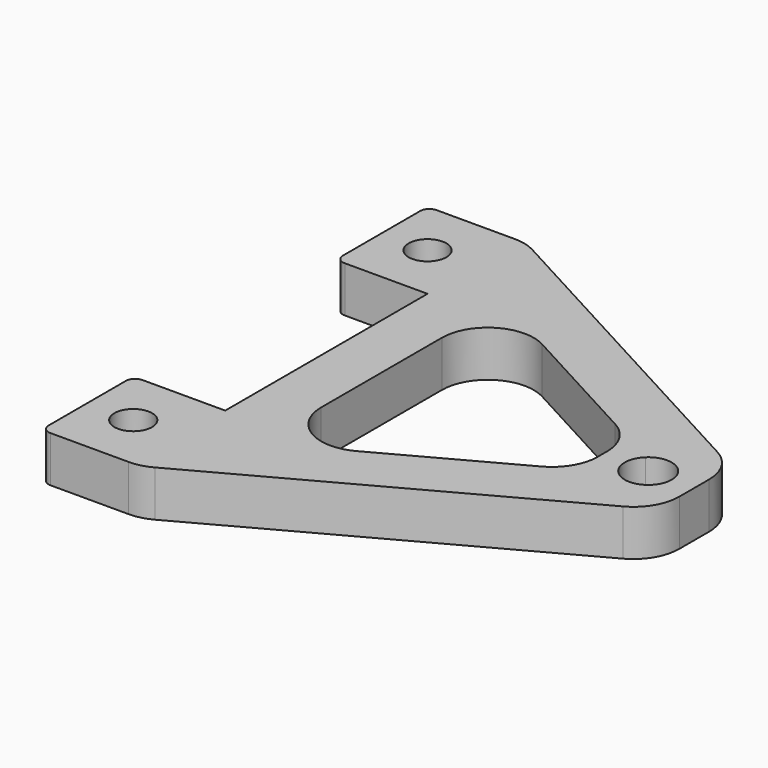
from build123d import *

# Parameters (mm, degrees)
F0_R     = 4.1
F1_DEPTH = 10
F2_R     = 10
F3_R     = 2


with BuildPart() as f1:
    # F0 (on Top) → F1 (new body)
    with BuildSketch(Plane.XY):
        Polygon((70, 30), (70, 40), (70, 50), (-8.4782754802, 92.5), (-30, 92.5), (-30, 67.5), (-10, 67.5), (-10, 12.5), (-30, 12.5), (-30, -12.5), (-8.4782754802, -12.5), align=None)
        with Locations((-20, 0)):
            Circle(F0_R, mode=Mode.SUBTRACT)
        with Locations((-20, 80)):
            Circle(F0_R, mode=Mode.SUBTRACT)
        with BuildLine():
            Line((2, 73.1787940384), (52.0543567222, 46.0717998075))
            ThreePointArc((52.0543567222, 46.0717998075), (63.2049623416, 49.472497896), (70, 40))
            ThreePointArc((70, 40), (63.2049623416, 30.527502104), (52.0543567222, 33.9282001925))
            Line((52.0543567222, 33.9282001925), (2, 6.8212059616))
            Line((2, 6.8212059616), (2, 73.1787940384))
        make_face(mode=Mode.SUBTRACT)
        with BuildLine():
            ThreePointArc((56.4697287247, 43.6806500408), (62.0007019388, 44.6911823405), (65.1, 40))
            ThreePointArc((65.1, 40), (62.0007019388, 35.3088176595), (56.4697287247, 36.3193499592))
            Line((56.4697287247, 36.3193499592), (52.0543567222, 33.9282001925))
            ThreePointArc((52.0543567222, 33.9282001925), (63.2049623416, 30.527502104), (70, 40))
            ThreePointArc((70, 40), (63.2049623416, 49.472497896), (52.0543567222, 46.0717998075))
            Line((52.0543567222, 46.0717998075), (56.4697287247, 43.6806500408))
        make_face()
        with BuildLine():
            ThreePointArc((56.4697287247, 36.3193499592), (54.9, 40), (56.4697287247, 43.6806500408))
            Line((56.4697287247, 43.6806500408), (52.0543567222, 46.0717998075))
            ThreePointArc((52.0543567222, 46.0717998075), (50, 40), (52.0543567222, 33.9282001925))
            Line((52.0543567222, 33.9282001925), (56.4697287247, 36.3193499592))
        make_face()
    extrude(amount=F1_DEPTH)

    # F2
    f2_edges = [f1.edges().sort_by_distance(p)[0] for p in [
        (-8.478275, 92.5, 5),
        (-8.478275, -12.5, 5),
        (70, 30, 5),
        (70, 50, 5),
        (52.054357, 46.0718, 5),
        (52.054357, 33.9282, 5),
        (2, 6.821206, 5),
        (2, 73.178794, 5),
    ]]
    fillet(f2_edges, radius=F2_R)

    # F3
    f3_edges = [f1.edges().sort_by_distance(p)[0] for p in [
        (-30, 92.5, 5),
        (-30, 67.5, 5),
        (-30, 12.5, 5),
        (-30, -12.5, 5),
    ]]
    fillet(f3_edges, radius=F3_R)


solid = f1.part
